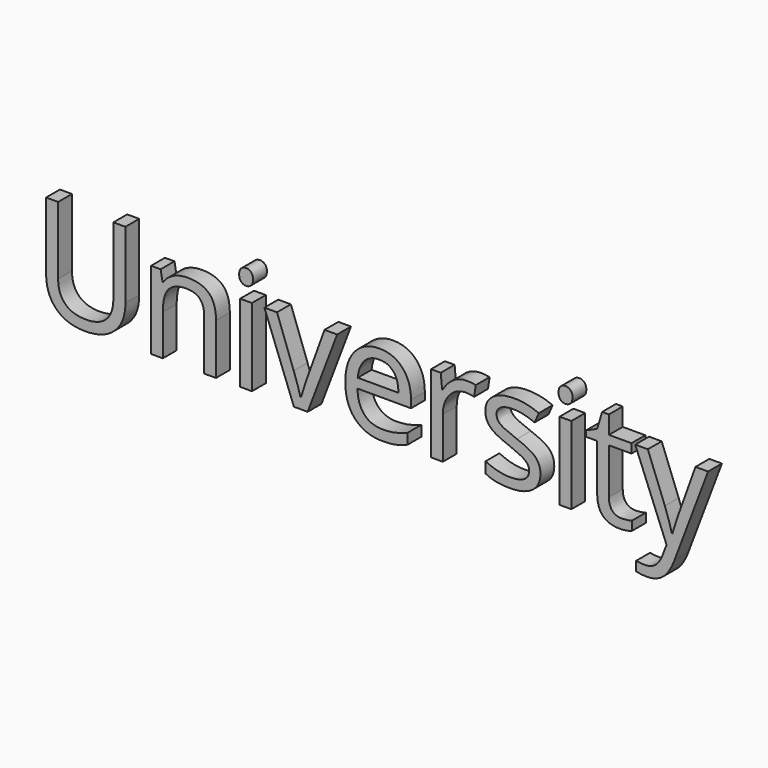
from build123d import *

# Parameters (mm, degrees)
F0_TEXT_SIZE = 213.2322949668
F1_DEPTH     = 25.4


# Not quite as in the source:
# - Text() gives the source's letters only with a copy of the font that has no kerning and outlines rounded to 1/6400 em; it was checked with that copy


with BuildPart() as f1:
    # F0 (on Front) → F1 (new body)
    with BuildSketch(Plane.XZ):
        with Locations((-75.2840265632, -76.6661763191)):
            Text('University', F0_TEXT_SIZE, font='Open Sans', text_align=(TextAlign.LEFT, TextAlign.BOTTOM))
    extrude(amount=F1_DEPTH)


solid = f1.part
